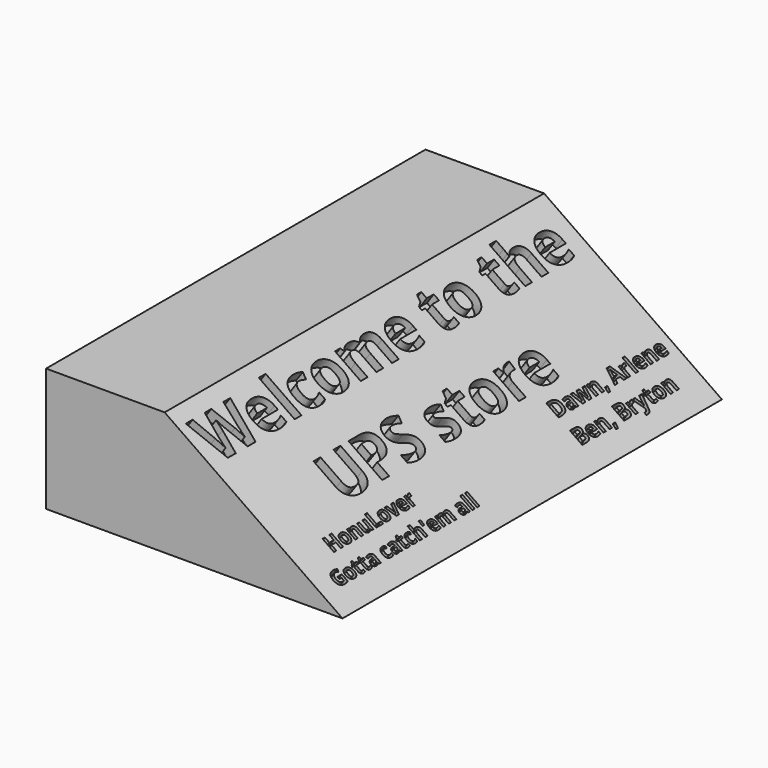
from build123d import *

# Parameters (mm, degrees)
F1_DEPTH       = 101.6
F2_TEXT_SIZE   = 12.3021528289
F2_TEXT_SIZE_2 = 4.5376133985
F2_TEXT_SIZE_3 = 4.1873883775
F3_DEPTH       = 2.54


# Not quite as in the source:
# - Text() gives the source's letters only with a copy of the font that has no kerning and outlines rounded to 1/6400 em; it was checked with that copy


with BuildPart() as f1:
    # F0 (on Front) → F1 (new body)
    with BuildSketch(Plane.XZ):
        Polygon((-24.6045703452, 0), (38.8954296548, 0), (0.7954296548, 26.4734386991), (-24.6045703452, 26.4734386991), align=None)
    extrude(amount=F1_DEPTH)

    # F2 (on face) → F3 (cut)
    with BuildSketch(Plane(origin=(12.6644291262, 0, 18.2263722968), x_dir=(0.8212173978, 0, -0.5706154446), z_dir=(0.5706154446, 0, 0.8212173978))):
        with Locations(Location((-2.1397956342, -99.5522447419), (0, 0, 90))):
            Text('Welcome to the', F2_TEXT_SIZE, font='Open Sans', font_style=FontStyle.BOLD, text_align=(TextAlign.LEFT, TextAlign.BOTTOM))
        with Locations(Location((14.5911322132, -83.5690571212), (0, 0, 90))):
            Text('UPS store', F2_TEXT_SIZE, font='Open Sans', font_style=FontStyle.BOLD, text_align=(TextAlign.LEFT, TextAlign.BOTTOM))
        with Locations(Location((20.4913059312, -32.3787631347), (0, 0, 90))):
            Text('Dawn, Arlene', F2_TEXT_SIZE_2, font='Open Sans', font_style=FontStyle.BOLD, text_align=(TextAlign.LEFT, TextAlign.BOTTOM))
        with Locations(Location((26.6624601531, -32.3787631347), (0, 0, 90))):
            Text('Ben, Bryton', F2_TEXT_SIZE_2, font='Open Sans', font_style=FontStyle.BOLD, text_align=(TextAlign.LEFT, TextAlign.BOTTOM))
        with Locations(Location((21.2267947427, -93.2565610693), (0, 0, 90))):
            Text('HonuLover', F2_TEXT_SIZE_3, font='Open Sans', font_style=FontStyle.BOLD, text_align=(TextAlign.LEFT, TextAlign.BOTTOM))
        with Locations(Location((26.9216429361, -97.6088278642), (0, 0, 90))):
            Text("Gotta catch'em all", F2_TEXT_SIZE_3, font='Open Sans', font_style=FontStyle.BOLD, text_align=(TextAlign.LEFT, TextAlign.BOTTOM))
    extrude(amount=-F3_DEPTH, mode=Mode.SUBTRACT)


solid = f1.part
